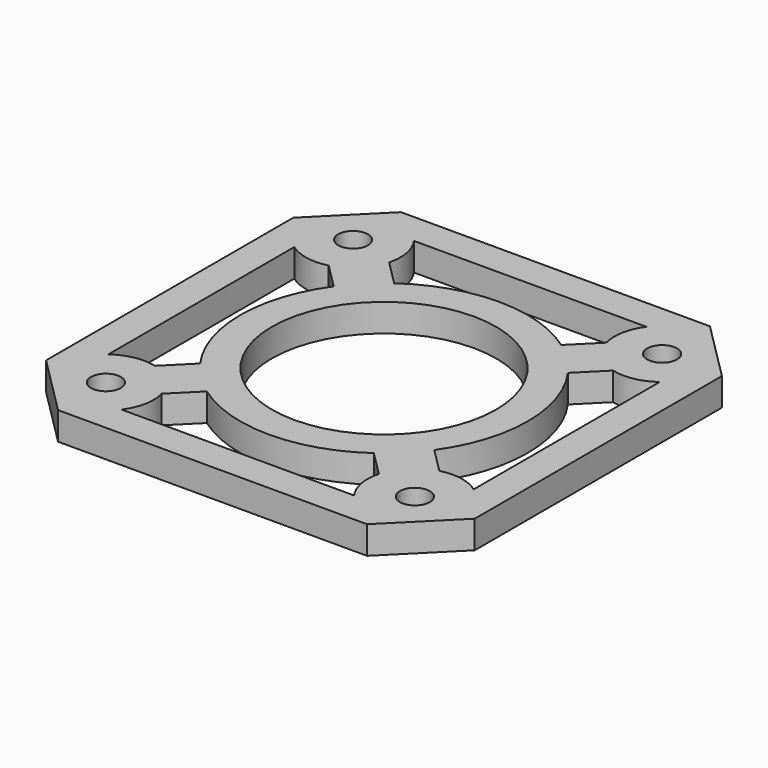
from build123d import *

# Parameters (mm, degrees)
F0_W            = 43.0059846
F0_H            = 43.0059846
F0_R            = 1.5
F0_R_2          = 11.2530001
F1_DEPTH        = 2.79375108
F2_SIZE         = 6.0030106
F4_DEPTH        = 2.79375108
F4_COPIES_COUNT = 4


# Not quite as in the source:
# - a pattern or mirror of a feature is missing from the dataset's text; its kind, count and spacing are read off the source's solid


with BuildPart() as f1:
    # F0 (on Top) → F1 (new body)
    with BuildSketch(Plane.XY):
        with Locations((21.5029923, 21.5029923)):
            Rectangle(F0_W, F0_H)
        with Locations((6.0029979, 6.0029979)):
            Circle(F0_R, mode=Mode.SUBTRACT)
        with Locations((21.5029923, 21.5029923)):
            Circle(F0_R_2, mode=Mode.SUBTRACT)
        with Locations((37.0029867, 6.0029979)):
            Circle(F0_R, mode=Mode.SUBTRACT)
        with Locations((6.0029979, 37.0029867)):
            Circle(F0_R, mode=Mode.SUBTRACT)
        with Locations((37.0029867, 37.0029867)):
            Circle(F0_R, mode=Mode.SUBTRACT)
    extrude(amount=F1_DEPTH)

    # F2
    f2_edges = [f1.edges().sort_by_distance(p)[0] for p in [
        (0, 0, 1.396876),
        (0, 43.005985, 1.396876),
        (43.005985, 0, 1.396876),
        (43.005985, 43.005985, 1.396876),
    ]]
    chamfer(f2_edges, length=F2_SIZE)

    # F3 (on face) → F4 (cut, through all)
    with BuildSketch(Plane.XY.offset(2.79375108)):
        with BuildLine():
            ThreePointArc((7.2356236023, 32.4027649523), (5.1176370603, 32.3235056996), (3.175, 33.171037571))
            Line((3.175, 33.171037571), (3.175, 9.834947029))
            ThreePointArc((3.175, 9.834947029), (5.1176370603, 10.6824789004), (7.2356236023, 10.6032196477))
            Line((7.2356236023, 10.6032196477), (9.7569670059, 13.1245630513))
            ThreePointArc((9.7569670059, 13.1245630513), (7.0749922, 21.5029923), (9.7569670059, 29.8814215487))
            Line((9.7569670059, 29.8814215487), (7.2356236023, 32.4027649523))
        make_face()
    f4 = extrude(amount=-F4_DEPTH, mode=Mode.SUBTRACT)

    # F4_copies: F4 ×4 about axis
    f4_copies_axis = Axis((21.502992, 21.502992, 0), (0, 0, 1))
    for i in range(1, F4_COPIES_COUNT):
        add(f4.rotate(f4_copies_axis, i * 360 / F4_COPIES_COUNT), mode=Mode.SUBTRACT)


solid = f1.part
